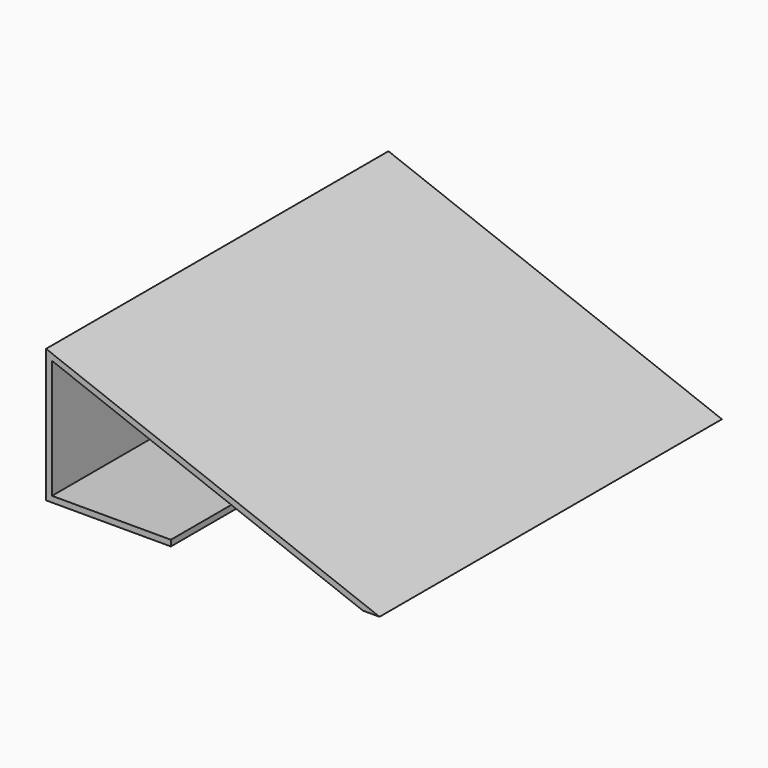
from build123d import *

# Parameters (mm, degrees)
F1_DEPTH = 457.2
F2_T     = 6.35
F3_W     = 205.1480994978
F3_H     = 457.2
F3_W_2   = 34.3874049749
F4_DEPTH = 6.35


with BuildPart() as f1:
    # F0 (on Front) → F1 (new body)
    with BuildSketch(Plane.XZ):
        Polygon((-127, 88.0205180943), (-127, -38.9794819057), (205.1480994978, -38.9794819057), align=None)
    extrude(amount=F1_DEPTH)

    # F2
    f2_openings = [f1.faces().sort_by_distance(p)[0] for p in [
        (-16.283967, -457.2, 3.353851),
        (-16.283967, 0, 3.353851),
    ]]
    offset(amount=F2_T, openings=f2_openings, kind=Kind.INTERSECTION)

    # F3 (on face) → F4 (cut)
    with BuildSketch(Plane(origin=(0, 0, -45.3294819057), x_dir=(1, 0, 0), z_dir=(0, 0, -1))):
        with Locations((102.5740497489, 228.6)):
            Rectangle(F3_W, F3_H)
        with Locations((222.3418019852, 228.6)):
            Rectangle(F3_W_2, F3_H)
    extrude(amount=-F4_DEPTH, mode=Mode.SUBTRACT)


solid = f1.part
